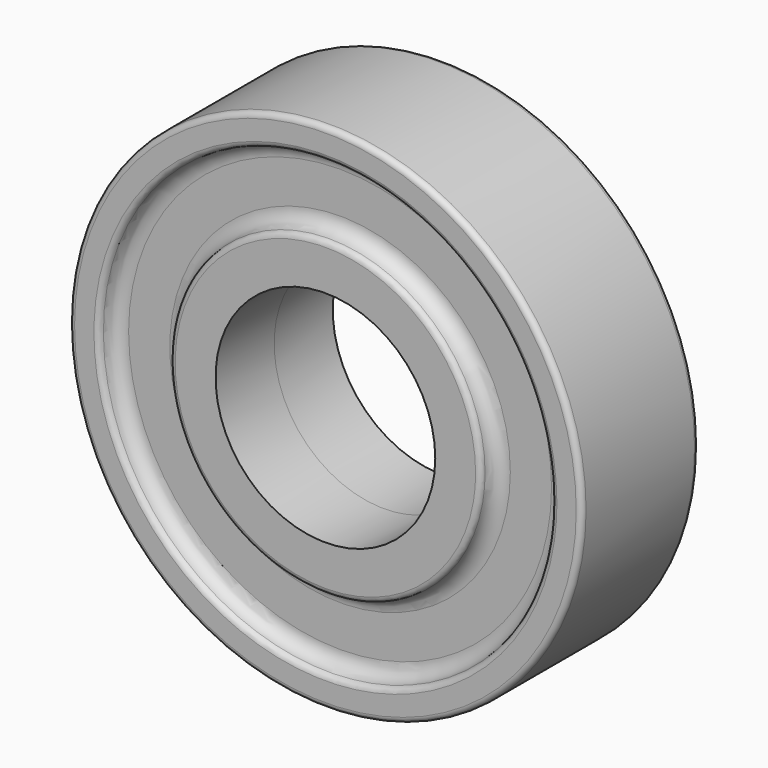
from build123d import *

# Parameters (mm, degrees)
F0_R          = 14
F0_R_2        = 6
F1_DEPTH      = 4
F1_DEPTH_BACK = 4
F2_R          = 12.35
F2_R_2        = 8.5
F3_DEPTH      = 1
F4_R          = 0.8
F5_R          = 0.3


# Not quite as in the source:
# - a pattern or mirror of a feature is missing from the dataset's text; its kind, count and spacing are read off the source's solid


with BuildPart() as f1:
    # F0 (on Front) → F1 (new body, two sides)
    with BuildSketch(Plane.XZ) as f1_sk:
        Circle(F0_R)
        Circle(F0_R_2, mode=Mode.SUBTRACT)
    extrude(amount=F1_DEPTH)
    extrude(f1_sk.sketch, amount=-F1_DEPTH_BACK)

    # F2 (on face) → F3 (cut)
    with BuildSketch(Plane.XZ.offset(4)):
        Circle(F2_R)
        Circle(F2_R_2, mode=Mode.SUBTRACT)
    f3 = extrude(amount=-F3_DEPTH, mode=Mode.SUBTRACT)

    # F3_copies: F3 across plane
    add(f3.mirror(Plane.ZX), mode=Mode.SUBTRACT)

    # F4
    f4_edges = [f1.edges().sort_by_distance(p)[0] for p in [
        (-8.5, -3, 0),
        (-12.35, -3, 0),
        (-12.35, 3, 0),
        (-8.5, 3, 0),
    ]]
    fillet(f4_edges, radius=F4_R)

    # F5
    f5_edges = [f1.edges().sort_by_distance(p)[0] for p in [
        (-12.35, -4, 0),
        (-14, -4, 0),
        (-8.5, -4, 0),
        (-14, 4, 0),
        (-12.35, 4, 0),
        (-8.5, 4, 0),
    ]]
    fillet(f5_edges, radius=F5_R)


solid = f1.part
